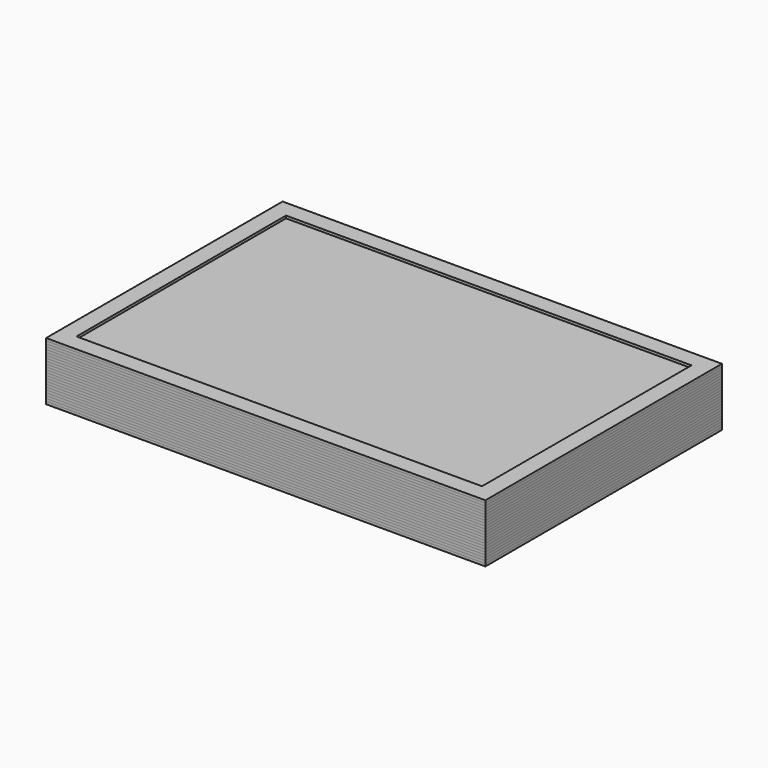
from build123d import *

# Parameters (mm, degrees)
F0_W      = 500
F0_H      = 330
F1_DEPTH  = 27
F2_W      = 347
F2_H      = 190
F3_DEPTH  = 35
F4_W      = 520
F4_H      = 350
F4_W_2    = 500
F4_H_2    = 330
F4_W_3    = 480
F4_H_3    = 310
F5_DEPTH  = 3
F7_DEPTH  = 3
F6_W      = 520
F6_H      = 350
F6_W_2    = 500
F6_H_2    = 330
F15_W     = 520
F15_H     = 350
F16_DEPTH = 3


# Not quite as in the source:
# - a feature names something its author has since deleted; it is built from what else it names


with BuildPart() as f1:
    # F0 (on Top) → F1 (new body)
    with BuildSketch(Plane.XY):
        Rectangle(F0_W, F0_H)
    extrude(amount=F1_DEPTH)

    # F2 (on face) → F3 (join)
    with BuildSketch(Plane(origin=(0, 0, 0), x_dir=(1, 0, 0), z_dir=(0, 0, -1))):
        with Locations((-3.5, 5)):
            Rectangle(F2_W, F2_H)
    extrude(amount=F3_DEPTH)


with BuildPart() as f5:
    # F4 (on face) → F5 (new body)
    with BuildSketch(Plane.XY.offset(27)):
        Rectangle(F4_W, F4_H)
        Rectangle(F4_W_2, F4_H_2, mode=Mode.SUBTRACT)
        Rectangle(F4_W_2, F4_H_2)
        Rectangle(F4_W_3, F4_H_3, mode=Mode.SUBTRACT)
    extrude(amount=F5_DEPTH)


with BuildPart() as f7:
    # F4 (on face) → F7 (new body)
    with BuildSketch(Plane.XY.offset(27)):
        Rectangle(F4_W, F4_H)
        Rectangle(F4_W_2, F4_H_2, mode=Mode.SUBTRACT)
    extrude(amount=-F7_DEPTH)


with BuildPart() as f7b:
    # F6 (on face) → F7, piece 2 (new body)
    with BuildSketch(Plane.XY.offset(27)):
        Rectangle(F6_W, F6_H)
        Rectangle(F6_W_2, F6_H_2, mode=Mode.SUBTRACT)
    extrude(amount=-F7_DEPTH)


with BuildPart() as f8_1:
    # F8: instance of F7b
    add(f7b.part.mirror(Plane(origin=(0, 0, 24), x_dir=(1, 0, 0), z_dir=(0, 0, -1))))


with BuildPart() as f9_1:
    # F9: instance of F8_1
    add(f8_1.part.mirror(Plane(origin=(0, 0, 21), x_dir=(1, 0, 0), z_dir=(0, 0, -1))))


with BuildPart() as f9_2:
    # F9: instance of F7
    add(f7.part.mirror(Plane(origin=(0, 0, 21), x_dir=(1, 0, 0), z_dir=(0, 0, -1))))


with BuildPart() as f10_1:
    # F10: instance of F9_2
    add(f9_2.part.mirror(Plane(origin=(0, 0, 15), x_dir=(1, 0, 0), z_dir=(0, 0, -1))))


with BuildPart() as f10_2:
    # F10: instance of F9_1
    add(f9_1.part.mirror(Plane(origin=(0, 0, 15), x_dir=(1, 0, 0), z_dir=(0, 0, -1))))


with BuildPart() as f10_3:
    # F10: instance of F8_1
    add(f8_1.part.mirror(Plane(origin=(0, 0, 15), x_dir=(1, 0, 0), z_dir=(0, 0, -1))))


with BuildPart() as f10_4:
    # F10: instance of F7
    add(f7.part.mirror(Plane(origin=(0, 0, 15), x_dir=(1, 0, 0), z_dir=(0, 0, -1))))


with BuildPart() as f11_1:
    # F11: instance of F10_4
    add(f10_4.part.mirror(Plane(origin=(0, 0, 3), x_dir=(1, 0, 0), z_dir=(0, 0, -1))))


with BuildPart() as f11_2:
    # F11: instance of F10_3
    add(f10_3.part.mirror(Plane(origin=(0, 0, 3), x_dir=(1, 0, 0), z_dir=(0, 0, -1))))


with BuildPart() as f11_3:
    # F11: instance of F10_2
    add(f10_2.part.mirror(Plane(origin=(0, 0, 3), x_dir=(1, 0, 0), z_dir=(0, 0, -1))))


with BuildPart() as f11_4:
    # F11: instance of F10_1
    add(f10_1.part.mirror(Plane(origin=(0, 0, 3), x_dir=(1, 0, 0), z_dir=(0, 0, -1))))


with BuildPart() as f11_5:
    # F11: instance of F9_2
    add(f9_2.part.mirror(Plane(origin=(0, 0, 3), x_dir=(1, 0, 0), z_dir=(0, 0, -1))))


with BuildPart() as f11_6:
    # F11: instance of F9_1
    add(f9_1.part.mirror(Plane(origin=(0, 0, 3), x_dir=(1, 0, 0), z_dir=(0, 0, -1))))


with BuildPart() as f11_7:
    # F11: instance of F8_1
    add(f8_1.part.mirror(Plane(origin=(0, 0, 3), x_dir=(1, 0, 0), z_dir=(0, 0, -1))))


with BuildPart() as f11_8:
    # F11: instance of F7
    add(f7.part.mirror(Plane(origin=(0, 0, 3), x_dir=(1, 0, 0), z_dir=(0, 0, -1))))


with BuildPart() as f12_1:
    # F12: instance of F11_8
    add(f11_8.part.mirror(Plane(origin=(0, 0, -21), x_dir=(1, 0, 0), z_dir=(0, 0, -1))))


with BuildPart() as f12_2:
    # F12: instance of F11_7
    add(f11_7.part.mirror(Plane(origin=(0, 0, -21), x_dir=(1, 0, 0), z_dir=(0, 0, -1))))


with BuildPart() as f12_3:
    # F12: instance of F11_6
    add(f11_6.part.mirror(Plane(origin=(0, 0, -21), x_dir=(1, 0, 0), z_dir=(0, 0, -1))))


with BuildPart() as f12_4:
    # F12: instance of F11_5
    add(f11_5.part.mirror(Plane(origin=(0, 0, -21), x_dir=(1, 0, 0), z_dir=(0, 0, -1))))


with BuildPart() as f12_5:
    # F12: instance of F11_4
    add(f11_4.part.mirror(Plane(origin=(0, 0, -21), x_dir=(1, 0, 0), z_dir=(0, 0, -1))))


with BuildPart() as f12_6:
    # F12: instance of F11_3
    add(f11_3.part.mirror(Plane(origin=(0, 0, -21), x_dir=(1, 0, 0), z_dir=(0, 0, -1))))


with BuildPart() as f12_7:
    # F12: instance of F11_1
    add(f11_1.part.mirror(Plane(origin=(0, 0, -21), x_dir=(1, 0, 0), z_dir=(0, 0, -1))))


with BuildPart() as f16:
    # F15 (on face) → F16 (new body)
    with BuildSketch(Plane(origin=(0, 0, -36), x_dir=(1, 0, 0), z_dir=(0, 0, -1))):
        Rectangle(F15_W, F15_H)
    extrude(amount=F16_DEPTH)


solid = Compound([f1.part, f5.part, f7.part, f7b.part, f8_1.part, f9_1.part, f9_2.part, f10_1.part, f10_2.part, f10_3.part, f10_4.part, f11_1.part, f11_2.part, f11_3.part, f11_4.part, f11_5.part, f11_6.part, f11_7.part, f11_8.part, f12_1.part, f12_2.part, f12_3.part, f12_4.part, f12_5.part, f16.part])
